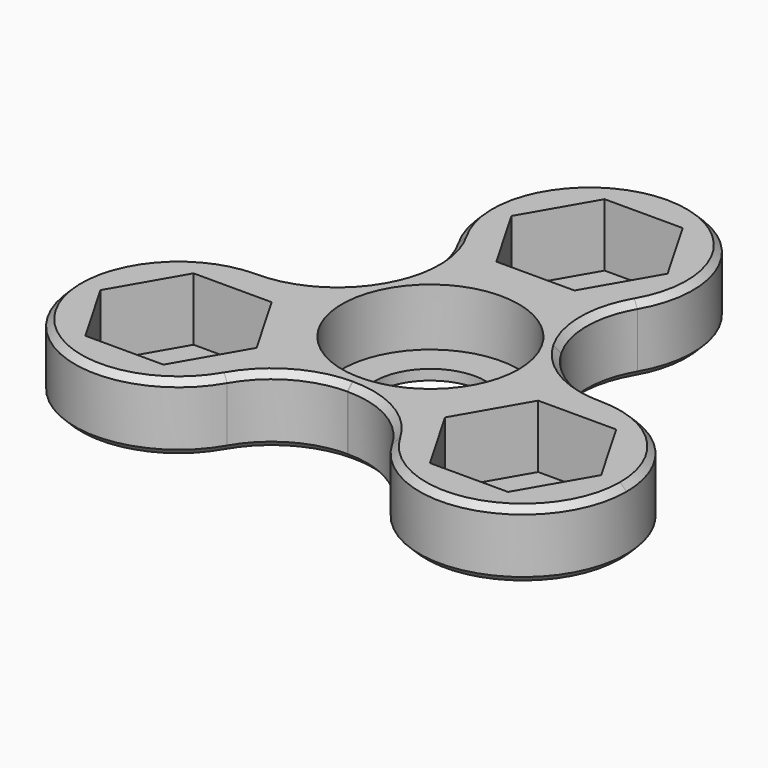
from build123d import *

# Parameters (mm, degrees)
F0_R     = 11.1
F0_R_2   = 7
F1_DEPTH = 0.6
F2_DEPTH = 8.5
F3_R     = 11.8527911282
F4_SIZE  = 0.8
F5_DEPTH = 1.3


# Not quite as in the source:
# - a feature names something its author has since deleted; it is built from what else it names


with BuildPart() as f1:
    # F0 (on Top) → F1 (new body)
    with BuildSketch(Plane.XY):
        with BuildLine():
            ThreePointArc((-3.5707142143, 12.5), (0, 13), (3.5707142143, 12.5))
            ThreePointArc((3.5707142143, 12.5), (10.3783256064, 17.1711841504), (13, 25))
            ThreePointArc((13, 25), (-7.8288158496, 35.3783256064), (-3.5707142143, 12.5))
        make_face()
        Polygon((4.9074772881, 33.5), (9.8149545762, 25), (4.9074772881, 16.5), (-4.9074772881, 16.5), (-9.8149545762, 25), (-4.9074772881, 33.5), align=None, mode=Mode.SUBTRACT)
        with BuildLine():
            ThreePointArc((-9.0399604402, -9.3423292192), (-11.2583302492, -6.5), (-12.6106746544, -3.1576707808))
            ThreePointArc((-12.6106746544, -3.1576707808), (-33.6197513051, -17.5734856991), (-8.6506350946, -12.5))
            ThreePointArc((-8.6506350946, -12.5), (-8.7483335459, -10.9092093959), (-9.0399604402, -9.3423292192))
        make_face()
        Polygon((-26.5581123827, -4), (-16.7431578065, -4), (-11.8356805184, -12.5), (-16.7431578065, -21), (-26.5581123827, -21), (-31.4655896708, -12.5), align=None, mode=Mode.SUBTRACT)
        with BuildLine():
            ThreePointArc((34.6506350946, -12.5), (26.7241207937, -0.5308837895), (12.6106746544, -3.1576707808))
            ThreePointArc((12.6106746544, -3.1576707808), (11.2583302492, -6.5), (9.0399604402, -9.3423292192))
            ThreePointArc((9.0399604402, -9.3423292192), (20.0598444905, -25.4023015487), (34.6506350946, -12.5))
        make_face()
        Polygon((16.7431578065, -21), (11.8356805184, -12.5), (16.7431578065, -4), (26.5581123827, -4), (31.4655896708, -12.5), (26.5581123827, -21), align=None, mode=Mode.SUBTRACT)
        with BuildLine():
            ThreePointArc((12.6106746544, -3.1576707808), (12.9023015487, -1.5907906041), (13, 0))
            ThreePointArc((13, 0), (10.3783256064, 7.8288158496), (3.5707142143, 12.5))
            ThreePointArc((3.5707142143, 12.5), (0, 12), (-3.5707142143, 12.5))
            ThreePointArc((-3.5707142143, 12.5), (-11.2583302492, 6.5), (-12.6106746544, -3.1576707808))
            ThreePointArc((-12.6106746544, -3.1576707808), (-10.3923048454, -6), (-9.0399604402, -9.3423292192))
            ThreePointArc((-9.0399604402, -9.3423292192), (0, -13), (9.0399604402, -9.3423292192))
            ThreePointArc((9.0399604402, -9.3423292192), (10.3923048454, -6), (12.6106746544, -3.1576707808))
        make_face()
        Circle(F0_R, mode=Mode.SUBTRACT)
        Circle(F0_R)
        Circle(F0_R_2, mode=Mode.SUBTRACT)
        Polygon((4.9074772881, 16.5), (9.8149545762, 25), (4.9074772881, 33.5), (-4.9074772881, 33.5), (-9.8149545762, 25), (-4.9074772881, 16.5), align=None)
        Polygon((-11.8356805184, -12.5), (-16.7431578065, -4), (-26.5581123827, -4), (-31.4655896708, -12.5), (-26.5581123827, -21), (-16.7431578065, -21), align=None)
        Polygon((16.7431578065, -4), (11.8356805184, -12.5), (16.7431578065, -21), (26.5581123827, -21), (31.4655896708, -12.5), (26.5581123827, -4), align=None)
        with BuildLine():
            ThreePointArc((-3.5707142143, 12.5), (0, 12), (3.5707142143, 12.5))
            ThreePointArc((3.5707142143, 12.5), (0, 13), (-3.5707142143, 12.5))
        make_face()
        with BuildLine():
            ThreePointArc((-9.0399604402, -9.3423292192), (-10.3923048454, -6), (-12.6106746544, -3.1576707808))
            ThreePointArc((-12.6106746544, -3.1576707808), (-11.2583302492, -6.5), (-9.0399604402, -9.3423292192))
        make_face()
        with BuildLine():
            ThreePointArc((9.0399604402, -9.3423292192), (11.2583302492, -6.5), (12.6106746544, -3.1576707808))
            ThreePointArc((12.6106746544, -3.1576707808), (10.3923048454, -6), (9.0399604402, -9.3423292192))
        make_face()
    extrude(amount=F1_DEPTH)

    # F0 (on Top) → F2 (join)
    with BuildSketch(Plane.XY):
        with BuildLine():
            ThreePointArc((-3.5707142143, 12.5), (0, 13), (3.5707142143, 12.5))
            ThreePointArc((3.5707142143, 12.5), (10.3783256064, 17.1711841504), (13, 25))
            ThreePointArc((13, 25), (-7.8288158496, 35.3783256064), (-3.5707142143, 12.5))
        make_face()
        Polygon((4.9074772881, 33.5), (9.8149545762, 25), (4.9074772881, 16.5), (-4.9074772881, 16.5), (-9.8149545762, 25), (-4.9074772881, 33.5), align=None, mode=Mode.SUBTRACT)
        with BuildLine():
            ThreePointArc((12.6106746544, -3.1576707808), (12.9023015487, -1.5907906041), (13, 0))
            ThreePointArc((13, 0), (10.3783256064, 7.8288158496), (3.5707142143, 12.5))
            ThreePointArc((3.5707142143, 12.5), (0, 12), (-3.5707142143, 12.5))
            ThreePointArc((-3.5707142143, 12.5), (-11.2583302492, 6.5), (-12.6106746544, -3.1576707808))
            ThreePointArc((-12.6106746544, -3.1576707808), (-10.3923048454, -6), (-9.0399604402, -9.3423292192))
            ThreePointArc((-9.0399604402, -9.3423292192), (0, -13), (9.0399604402, -9.3423292192))
            ThreePointArc((9.0399604402, -9.3423292192), (10.3923048454, -6), (12.6106746544, -3.1576707808))
        make_face()
        Circle(F0_R, mode=Mode.SUBTRACT)
        with BuildLine():
            ThreePointArc((-3.5707142143, 12.5), (0, 12), (3.5707142143, 12.5))
            ThreePointArc((3.5707142143, 12.5), (0, 13), (-3.5707142143, 12.5))
        make_face()
        with BuildLine():
            ThreePointArc((-9.0399604402, -9.3423292192), (-11.2583302492, -6.5), (-12.6106746544, -3.1576707808))
            ThreePointArc((-12.6106746544, -3.1576707808), (-33.6197513051, -17.5734856991), (-8.6506350946, -12.5))
            ThreePointArc((-8.6506350946, -12.5), (-8.7483335459, -10.9092093959), (-9.0399604402, -9.3423292192))
        make_face()
        Polygon((-26.5581123827, -4), (-16.7431578065, -4), (-11.8356805184, -12.5), (-16.7431578065, -21), (-26.5581123827, -21), (-31.4655896708, -12.5), align=None, mode=Mode.SUBTRACT)
        with BuildLine():
            ThreePointArc((-9.0399604402, -9.3423292192), (-10.3923048454, -6), (-12.6106746544, -3.1576707808))
            ThreePointArc((-12.6106746544, -3.1576707808), (-11.2583302492, -6.5), (-9.0399604402, -9.3423292192))
        make_face()
        with BuildLine():
            ThreePointArc((34.6506350946, -12.5), (26.7241207937, -0.5308837895), (12.6106746544, -3.1576707808))
            ThreePointArc((12.6106746544, -3.1576707808), (11.2583302492, -6.5), (9.0399604402, -9.3423292192))
            ThreePointArc((9.0399604402, -9.3423292192), (20.0598444905, -25.4023015487), (34.6506350946, -12.5))
        make_face()
        Polygon((16.7431578065, -21), (11.8356805184, -12.5), (16.7431578065, -4), (26.5581123827, -4), (31.4655896708, -12.5), (26.5581123827, -21), align=None, mode=Mode.SUBTRACT)
        with BuildLine():
            ThreePointArc((9.0399604402, -9.3423292192), (11.2583302492, -6.5), (12.6106746544, -3.1576707808))
            ThreePointArc((12.6106746544, -3.1576707808), (10.3923048454, -6), (9.0399604402, -9.3423292192))
        make_face()
    extrude(amount=F2_DEPTH)

    # F3
    f3_edges = [f1.edges().sort_by_distance(p)[0] for p in [
        (3.570714, 12.5, 4.25),
        (-3.570714, 12.5, 4.25),
        (-12.610675, -3.157671, 4.25),
        (-9.03996, -9.342329, 4.25),
        (9.03996, -9.342329, 4.25),
        (12.610675, -3.157671, 4.25),
    ]]
    fillet(f3_edges, radius=F3_R)

    # F4
    f4_edges = [f1.edges().sort_by_distance(p)[0] for p in [
        (11.25833, 6.5, 8.5),
        (9.627694, 12.5, 8.5),
        (0, 38, 8.5),
        (-9.627694, 12.5, 8.5),
        (-11.25833, 6.5, 8.5),
        (-11.25833, 6.5, 0),
        (-9.627694, 12.5, 0),
        (0, 38, 0),
        (9.627694, 12.5, 0),
        (11.25833, 6.5, 0),
        (15.639164, 2.087827, 8.5),
        (-15.639164, 2.087827, 8.5),
        (32.908965, -19, 8.5),
        (-32.908965, -19, 8.5),
        (6.011471, -14.587827, 8.5),
        (-6.011471, -14.587827, 8.5),
        (0, -13, 8.5),
        (15.639164, 2.087827, 0),
        (-15.639164, 2.087827, 0),
        (32.908965, -19, 0),
        (-32.908965, -19, 0),
        (6.011471, -14.587827, 0),
        (-6.011471, -14.587827, 0),
        (0, -13, 0),
    ]]
    chamfer(f4_edges, length=F4_SIZE)

    # F0 (on Top) → F5 (join)
    with BuildSketch(Plane.XY):
        Circle(F0_R)
        Circle(F0_R_2, mode=Mode.SUBTRACT)
    extrude(amount=F5_DEPTH)


solid = f1.part
